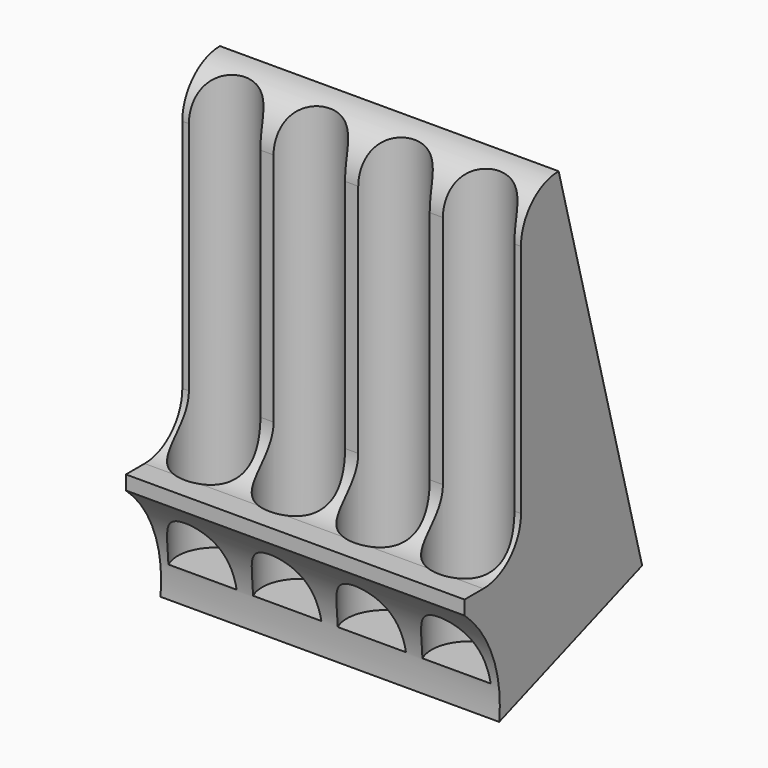
from build123d import *

# Parameters (mm, degrees)
F0_W         = 72
F0_H         = 100
F1_DEPTH     = 25
F2_R         = 8
F3_DEPTH     = 90
F4_W         = 72
F4_H         = 15
F5_DEPTH     = 70
F6_T4_DEPTH  = 26.4006579232
F6_S5_R      = 8
F6_T6_DEPTH  = 16
F6_S7_R      = 8
F6_T8_DEPTH  = 16
F6_T12_DEPTH = 52.8013158464
F6_S13_R     = 8
F6_T14_DEPTH = 29
F6_S15_R     = 8
F6_T16_DEPTH = 29
F6_S17_R     = 8
F6_T18_DEPTH = 29
F6_T23_DEPTH = 52.8013158464
F6_S24_R     = 8
F6_T25_DEPTH = 29
F6_S26_R     = 8
F6_T27_DEPTH = 29
F6_S28_R     = 8
F6_T29_DEPTH = 29
F6_S30_R     = 8
F6_T31_DEPTH = 29
F6_T35_DEPTH = 52.8013158464
F6_S36_R     = 8
F6_T37_DEPTH = 29
F6_S38_R     = 8
F6_T39_DEPTH = 29
F6_S40_R     = 8
F6_T41_DEPTH = 29
F6_T46_DEPTH = 26.4006579232
F6_S47_R     = 8
F6_T48_DEPTH = 16
F6_S49_R     = 8
F6_T50_DEPTH = 16
F6_T51_DEPTH = 51.4006579232
F6_T53_DEPTH = 52.8013158464
F6_T55_DEPTH = 52.8013158464
F6_T57_DEPTH = 52.8013158464
F6_T59_DEPTH = 51.4006579232
F8_DEPTH     = 72.0010001
F10_DEPTH    = 72.0010001
F12_DEPTH    = 72


# Not quite as in the source:
# - a fillet or chamfer that OpenCascade refuses, or shapes differently, is made with other operations: its cross-section is extruded or revolved along the edge and cut away or added


with BuildPart() as f1:
    # F0 (on Front) → F1 (new body)
    with BuildSketch(Plane.XZ):
        Rectangle(F0_W, F0_H)
    extrude(amount=-F1_DEPTH)

    # F2 (on face) → F3 (cut)
    with BuildSketch(Plane.XY.offset(50)):
        with Locations((-27, 12.5)):
            Circle(F2_R)
        with Locations((-9, 12.5)):
            Circle(F2_R)
        with Locations((9, 12.5)):
            Circle(F2_R)
        with Locations((27, 12.5)):
            Circle(F2_R)
    extrude(amount=-F3_DEPTH, mode=Mode.SUBTRACT)

    # F4 (on face) → F5 (cut)
    with BuildSketch(Plane.XY.offset(50)):
        with Locations((0, 7.5)):
            Rectangle(F4_W, F4_H)
    extrude(amount=-F5_DEPTH, mode=Mode.SUBTRACT)

    # F6: fillet of radius 10 on 10 edges, made by hand


with BuildPart() as f6_tool2:
    # F6_s3 → F6_t4 (new body)
    with BuildSketch(Plane.YZ.offset(-9.5993420768)):
        with BuildLine():
            ThreePointArc((15, -10), (12.0710678119, -17.0710678119), (5, -20))
            Line((5, -20), (15, -20))
            Line((15, -20), (15, -10))
        make_face()
    extrude(amount=-F6_T4_DEPTH)

    # F6_s5 → F6_t6 (cut, symmetric)
    with BuildSketch(Plane.XY.offset(-15)):
        with Locations((-9, 12.5)):
            Circle(F6_S5_R)
    extrude(amount=F6_T6_DEPTH, both=True, mode=Mode.SUBTRACT)

    # F6_s7 → F6_t8 (cut, symmetric)
    with BuildSketch(Plane.XY.offset(-15)):
        with Locations((-27, 12.5)):
            Circle(F6_S7_R)
    extrude(amount=F6_T8_DEPTH, both=True, mode=Mode.SUBTRACT)


with BuildPart() as f1_1:
    add(f1.part)

    # F6_t1: union F6_tool2
    add(f6_tool2.part)


with BuildPart() as f6_tool10:
    # F6_s11 → F6_t12 (new body)
    with BuildSketch(Plane.YZ.offset(8.4006579232)):
        with BuildLine():
            ThreePointArc((15, -10), (12.0710678119, -17.0710678119), (5, -20))
            Line((5, -20), (15, -20))
            Line((15, -20), (15, -10))
        make_face()
    extrude(amount=-F6_T12_DEPTH)

    # F6_s13 → F6_t14 (cut, symmetric)
    with BuildSketch(Plane.XY.offset(-15)):
        with Locations((9, 12.5)):
            Circle(F6_S13_R)
    extrude(amount=F6_T14_DEPTH, both=True, mode=Mode.SUBTRACT)

    # F6_s15 → F6_t16 (cut, symmetric)
    with BuildSketch(Plane.XY.offset(-15)):
        with Locations((-9, 12.5)):
            Circle(F6_S15_R)
    extrude(amount=F6_T16_DEPTH, both=True, mode=Mode.SUBTRACT)

    # F6_s17 → F6_t18 (cut, symmetric)
    with BuildSketch(Plane.XY.offset(-15)):
        with Locations((-27, 12.5)):
            Circle(F6_S17_R)
    extrude(amount=F6_T18_DEPTH, both=True, mode=Mode.SUBTRACT)

    split(bisect_by=Plane.YZ.offset(-36), keep=Keep.TOP)


with BuildPart() as f1_2:
    add(f1_1.part)

    # F6_t9: union F6_tool10
    add(f6_tool10.part)


with BuildPart() as f6_tool21:
    # F6_s22 → F6_t23 (new body)
    with BuildSketch(Plane.YZ.offset(26.4006579232)):
        with BuildLine():
            ThreePointArc((15, -10), (12.0710678119, -17.0710678119), (5, -20))
            Line((5, -20), (15, -20))
            Line((15, -20), (15, -10))
        make_face()
    extrude(amount=-F6_T23_DEPTH)

    # F6_s24 → F6_t25 (cut, symmetric)
    with BuildSketch(Plane.XY.offset(-15)):
        with Locations((27, 12.5)):
            Circle(F6_S24_R)
    extrude(amount=F6_T25_DEPTH, both=True, mode=Mode.SUBTRACT)

    # F6_s26 → F6_t27 (cut, symmetric)
    with BuildSketch(Plane.XY.offset(-15)):
        with Locations((9, 12.5)):
            Circle(F6_S26_R)
    extrude(amount=F6_T27_DEPTH, both=True, mode=Mode.SUBTRACT)

    # F6_s28 → F6_t29 (cut, symmetric)
    with BuildSketch(Plane.XY.offset(-15)):
        with Locations((-9, 12.5)):
            Circle(F6_S28_R)
    extrude(amount=F6_T29_DEPTH, both=True, mode=Mode.SUBTRACT)

    # F6_s30 → F6_t31 (cut, symmetric)
    with BuildSketch(Plane.XY.offset(-15)):
        with Locations((-27, 12.5)):
            Circle(F6_S30_R)
    extrude(amount=F6_T31_DEPTH, both=True, mode=Mode.SUBTRACT)


with BuildPart() as f1_3:
    add(f1_2.part)

    # F6_t20: union F6_tool21
    add(f6_tool21.part)


with BuildPart() as f6_tool33:
    # F6_s34 → F6_t35 (new body)
    with BuildSketch(Plane.YZ.offset(44.4006579232)):
        with BuildLine():
            ThreePointArc((15, -10), (12.0710678119, -17.0710678119), (5, -20))
            Line((5, -20), (15, -20))
            Line((15, -20), (15, -10))
        make_face()
    extrude(amount=-F6_T35_DEPTH)

    # F6_s36 → F6_t37 (cut, symmetric)
    with BuildSketch(Plane.XY.offset(-15)):
        with Locations((27, 12.5)):
            Circle(F6_S36_R)
    extrude(amount=F6_T37_DEPTH, both=True, mode=Mode.SUBTRACT)

    # F6_s38 → F6_t39 (cut, symmetric)
    with BuildSketch(Plane.XY.offset(-15)):
        with Locations((9, 12.5)):
            Circle(F6_S38_R)
    extrude(amount=F6_T39_DEPTH, both=True, mode=Mode.SUBTRACT)

    # F6_s40 → F6_t41 (cut, symmetric)
    with BuildSketch(Plane.XY.offset(-15)):
        with Locations((-9, 12.5)):
            Circle(F6_S40_R)
    extrude(amount=F6_T41_DEPTH, both=True, mode=Mode.SUBTRACT)

    split(bisect_by=Plane.YZ.offset(36), keep=Keep.BOTTOM)


with BuildPart() as f1_4:
    add(f1_3.part)

    # F6_t32: union F6_tool33
    add(f6_tool33.part)


with BuildPart() as f6_tool44:
    # F6_s45 → F6_t46 (new body)
    with BuildSketch(Plane.YZ.offset(36)):
        with BuildLine():
            ThreePointArc((15, -10), (12.0710678119, -17.0710678119), (5, -20))
            Line((5, -20), (15, -20))
            Line((15, -20), (15, -10))
        make_face()
    extrude(amount=-F6_T46_DEPTH)

    # F6_s47 → F6_t48 (cut, symmetric)
    with BuildSketch(Plane.XY.offset(-15)):
        with Locations((27, 12.5)):
            Circle(F6_S47_R)
    extrude(amount=F6_T48_DEPTH, both=True, mode=Mode.SUBTRACT)

    # F6_s49 → F6_t50 (cut, symmetric)
    with BuildSketch(Plane.XY.offset(-15)):
        with Locations((9, 12.5)):
            Circle(F6_S49_R)
    extrude(amount=F6_T50_DEPTH, both=True, mode=Mode.SUBTRACT)


with BuildPart() as f1_5:
    add(f1_4.part)

    # F6_t43: union F6_tool44
    add(f6_tool44.part)

    # F6_s52 → F6_t51 (cut)
    with BuildSketch(Plane.YZ.offset(-61)):
        with BuildLine():
            ThreePointArc((25, 50), (17.9289321881, 47.0710678119), (15, 40))
            Line((15, 40), (15, 50))
            Line((15, 50), (25, 50))
        make_face()
    extrude(amount=F6_T51_DEPTH, mode=Mode.SUBTRACT)

    # F6_s54 → F6_t53 (cut)
    with BuildSketch(Plane.YZ.offset(-44.4006579232)):
        with BuildLine():
            ThreePointArc((25, 50), (17.9289321881, 47.0710678119), (15, 40))
            Line((15, 40), (15, 50))
            Line((15, 50), (25, 50))
        make_face()
    extrude(amount=F6_T53_DEPTH, mode=Mode.SUBTRACT)

    # F6_s56 → F6_t55 (cut)
    with BuildSketch(Plane.YZ.offset(-26.4006579232)):
        with BuildLine():
            ThreePointArc((25, 50), (17.9289321881, 47.0710678119), (15, 40))
            Line((15, 40), (15, 50))
            Line((15, 50), (25, 50))
        make_face()
    extrude(amount=F6_T55_DEPTH, mode=Mode.SUBTRACT)

    # F6_s58 → F6_t57 (cut)
    with BuildSketch(Plane.YZ.offset(-8.4006579232)):
        with BuildLine():
            ThreePointArc((25, 50), (17.9289321881, 47.0710678119), (15, 40))
            Line((15, 40), (15, 50))
            Line((15, 50), (25, 50))
        make_face()
    extrude(amount=F6_T57_DEPTH, mode=Mode.SUBTRACT)

    # F6_s60 → F6_t59 (cut)
    with BuildSketch(Plane.YZ.offset(9.5993420768)):
        with BuildLine():
            ThreePointArc((25, 50), (17.9289321881, 47.0710678119), (15, 40))
            Line((15, 40), (15, 50))
            Line((15, 50), (25, 50))
        make_face()
    extrude(amount=F6_T59_DEPTH, mode=Mode.SUBTRACT)

    # F7 (on face) → F8 (cut, through all)
    with BuildSketch(Plane.YZ.offset(36)):
        Polygon((25, -40.9007441433), (0, -50), (25, -50), align=None)
    extrude(amount=-F8_DEPTH, mode=Mode.SUBTRACT)

    # F9 (on face) → F10 (cut, through all)
    with BuildSketch(Plane.YZ.offset(36)):
        with BuildLine():
            Line((0, -50), (9.2097919016, -46.647909884))
            ThreePointArc((9.2097919016, -46.647909884), (7.5034777784, -33.6953798419), (0, -23.0006445199))
            Line((0, -23.0006445199), (0, -50))
        make_face()
    extrude(amount=-F10_DEPTH, mode=Mode.SUBTRACT)

    # F11 (on face) → F12 (join)
    with BuildSketch(Plane.YZ.offset(36)):
        Polygon((25, 50), (25, -40.9007441433), (47.1924504818, -32.8233527425), align=None)
    extrude(amount=-F12_DEPTH)


solid = f1_5.part
